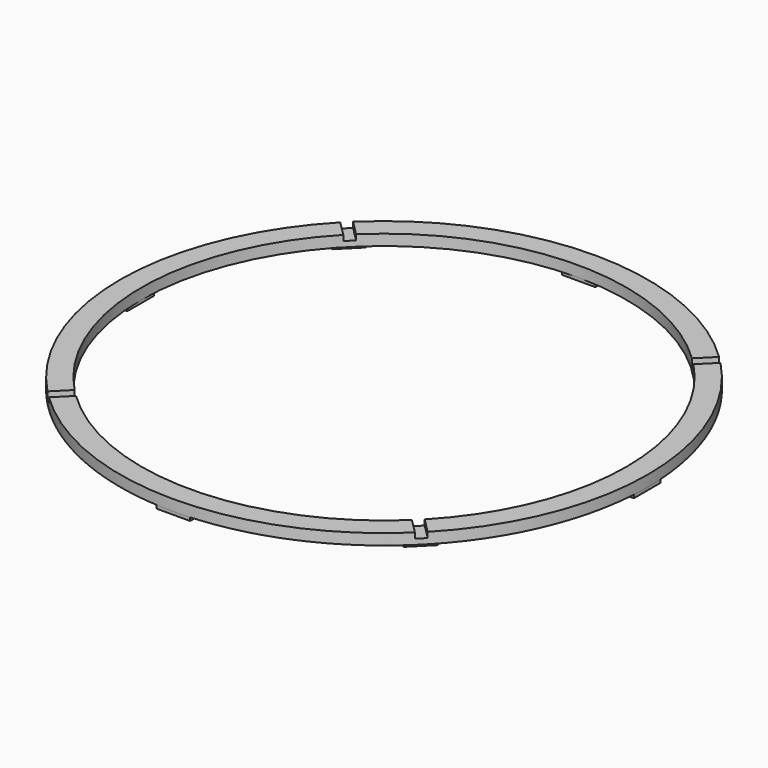
from build123d import *

# Parameters (mm, degrees)
F0_R            = 78.74
F0_R_2          = 72.39
F1_DEPTH        = 3.25
F3_DEPTH        = 1.63
F3_COPIES_COUNT = 4
F6_DEPTH        = 1
F7_COUNT        = 4
F7_ANGLE        = 270
F9_DEPTH        = 1
F10_COUNT       = 4
F10_ANGLE       = 270


# Not quite as in the source:
# - a feature of the source that left no trace in its solid (it failed there, or was rolled back) is left out
# - a pattern or mirror of a feature is missing from the dataset's text; its kind, count and spacing are read off the source's solid


with BuildPart() as f1:
    # F0 (on Top) → F1 (new body)
    with BuildSketch(Plane.XY):
        Circle(F0_R)
        Circle(F0_R_2, mode=Mode.SUBTRACT)
    extrude(amount=F1_DEPTH)

    # F2 (on face) → F3 (cut)
    with BuildSketch(Plane.XY.offset(3.25)):
        with BuildLine():
            Line((-50.1158095189, 52.2371298624), (-54.6068240538, 56.7281443973))
            ThreePointArc((-54.6068240538, 56.7281443973), (-55.6775879506, 55.6775879506), (-56.7281443973, 54.6068240538))
            Line((-56.7281443973, 54.6068240538), (-52.2371298624, 50.1158095189))
            ThreePointArc((-52.2371298624, 50.1158095189), (-51.1874598901, 51.1874598901), (-50.1158095189, 52.2371298624))
        make_face()
    f3 = extrude(amount=-F3_DEPTH, mode=Mode.SUBTRACT)

    # F3_copies: F3 ×4 about axis
    f3_copies_axis = Axis((0, 0, 0), (0, 0, 1))
    for i in range(1, F3_COPIES_COUNT):
        add(f3.rotate(f3_copies_axis, i * 360 / F3_COPIES_COUNT), mode=Mode.SUBTRACT)

    # F5 (on face) → F6 (join)
    with BuildSketch(Plane(origin=(0, 0, 0), x_dir=(1, 0, 0), z_dir=(0, 0, -1))):
        Polygon((-54.8467374827, 49.1898832332), (-52.018310358, 52.018310358), (-54.8467374827, 54.8467374827), (-57.6751646075, 52.018310358), (-56.2609510451, 50.6040967956), align=None)
        Polygon((-54.8467374827, 54.8467374827), (-52.018310358, 52.018310358), (-49.1898832332, 54.8467374827), (-50.6040967956, 56.2609510451), (-52.018310358, 57.6751646075), align=None)
    f6 = extrude(amount=F6_DEPTH)

    # F7: F6 ×4 about axis
    f7_axis = Axis((0, 0, 0), (0, 0, -1))
    for i in range(1, F7_COUNT):
        add(f6.rotate(f7_axis, i * F7_ANGLE / (F7_COUNT - 1)))

    # F8 (on face) → F9 (join)
    with BuildSketch(Plane(origin=(0, 0, 0), x_dir=(1, 0, 0), z_dir=(0, 0, -1))):
        Polygon((-5, 78.565), (-5, 75.565), (-5, 72.565), (0, 72.565), (5, 72.565), (5, 75.565), (5, 78.565), (0, 78.565), align=None)
    f9 = extrude(amount=F9_DEPTH)

    # F10: F9 ×4 about axis
    f10_axis = Axis((0, 0, 0), (0, 0, 1))
    for i in range(1, F10_COUNT):
        add(f9.rotate(f10_axis, i * F10_ANGLE / (F10_COUNT - 1)))


solid = f1.part
